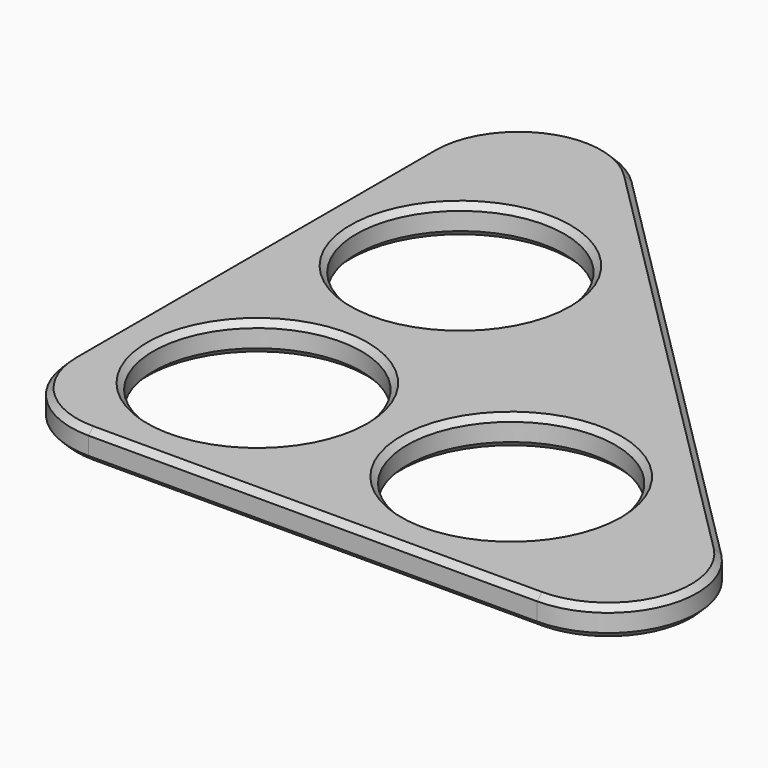
from build123d import *

# Parameters (mm, degrees)
F0_R     = 17.5846989279
F1_DEPTH = 5
F2_R     = 15
F3_SIZE  = 1


# Not quite as in the source:
# - a feature names something its author has since deleted; it is built from what else it names


with BuildPart() as f1:
    # F0 (on Top) → F1 (new body)
    with BuildSketch(Plane.XY):
        Polygon((0, 127), (0, 0), (127, 0), align=None)
        with Locations((24.1695605218, 24.1695605218)):
            Circle(F0_R, mode=Mode.SUBTRACT)
        with Locations((67.0569464564, 24.1695605218)):
            Circle(F0_R, mode=Mode.SUBTRACT)
        with Locations((24.1695605218, 67.0569464564)):
            Circle(F0_R, mode=Mode.SUBTRACT)
    extrude(amount=F1_DEPTH)

    # F2
    f2_edges = [f1.edges().sort_by_distance(p)[0] for p in [
        (127, 0, 2.5),
        (0, 0, 2.5),
        (0, 127, 2.5),
    ]]
    fillet(f2_edges, radius=F2_R)

    # F3
    f3_edges = [f1.edges().sort_by_distance(p)[0] for p in [
        (104.64499, 9.259749, 5),
        (63.5, 63.5, 0),
        (6.584862, 24.169561, 5),
        (49.472248, 24.169561, 5),
        (6.584862, 67.056946, 0),
        (6.584862, 24.169561, 0),
        (49.472248, 24.169561, 0),
        (6.584862, 67.056946, 5),
        (0, 52.893398, 0),
        (0, 52.893398, 5),
        (9.259749, 104.64499, 0),
        (4.393398, 4.393398, 0),
        (52.893398, 0, 0),
        (104.64499, 9.259749, 0),
        (9.259749, 104.64499, 5),
        (4.393398, 4.393398, 5),
        (63.5, 63.5, 5),
        (52.893398, 0, 5),
    ]]
    chamfer(f3_edges, length=F3_SIZE)


solid = f1.part
